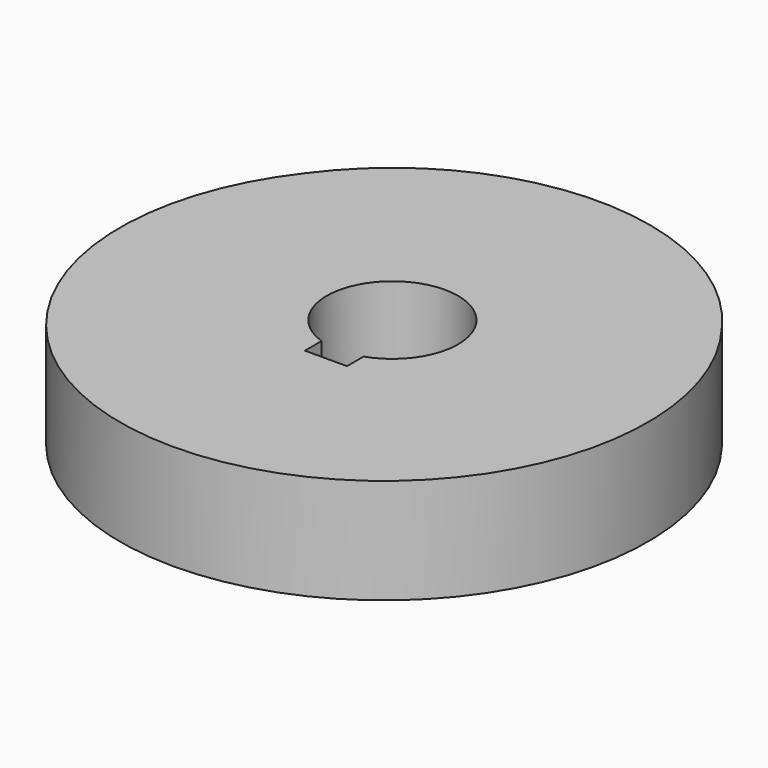
from build123d import *

# Parameters (mm, degrees)
F1_DEPTH = 200
F3_DEPTH = 469.9


# Not quite as in the source:
# - a feature names something its author has since deleted; it is built from what else it names


with BuildPart() as f1:
    # F0 (on Top) → F1 (new body)
    with BuildSketch(Plane.XY):
        with BuildLine():
            ThreePointArc((-396.7193466419, 287.6), (-151.1746012819, -466.0968138995), (490, 0))
            ThreePointArc((490, 0), (466.0968138995, 151.1746012818), (396.7193466419, 287.6))
            ThreePointArc((396.7193466419, 287.6), (0, 482), (-396.7193466419, 287.6))
        make_face()
        with BuildLine():
            ThreePointArc((396.7193466419, 287.6), (466.0968138995, 151.1746012818), (490, 0))
            ThreePointArc((490, 0), (-151.1746012819, -466.0968138995), (-396.7193466419, 287.6))
            ThreePointArc((-396.7193466419, 287.6), (-162.5590477115, -494.9511090703), (502, -20))
            ThreePointArc((502, -20), (474.9511090703, 142.5590477115), (396.7193466419, 287.6))
        make_face()
        with BuildLine():
            ThreePointArc((-396.7193466419, 287.6), (0, 482), (396.7193466419, 287.6))
            ThreePointArc((396.7193466419, 287.6), (0, 490), (-396.7193466419, 287.6))
        make_face()
    extrude(amount=-F1_DEPTH)

    # F2 (on Top) → F3 (cut)
    with BuildSketch(Plane.XY):
        with BuildLine():
            ThreePointArc((40, -118.4271928233), (101.5504800579, -72.8868986856), (125, 0))
            ThreePointArc((125, 0), (-72.8868986856, 101.5504800579), (-40, -118.4271928233))
            Line((-40, -118.4271928233), (-40, 0))
            Line((-40, 0), (40, 0))
            Line((40, 0), (40, -118.4271928233))
        make_face()
        with BuildLine():
            Line((-40, 0), (-40, -118.4271928233))
            ThreePointArc((-40, -118.4271928233), (0, -125), (40, -118.4271928233))
            Line((40, -118.4271928233), (40, 0))
            Line((40, 0), (-40, 0))
        make_face()
        with BuildLine():
            ThreePointArc((40, -118.4271928233), (0, -125), (-40, -118.4271928233))
            Line((-40, -118.4271928233), (-40, -158))
            Line((-40, -158), (40, -158))
            Line((40, -158), (40, -118.4271928233))
        make_face()
    extrude(amount=-F3_DEPTH, mode=Mode.SUBTRACT)


solid = f1.part
